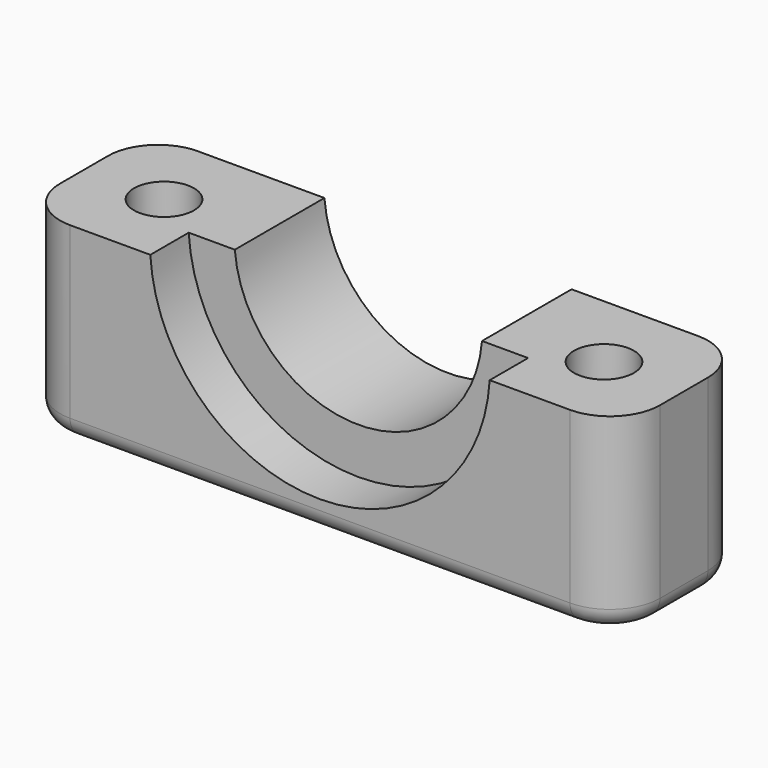
from build123d import *

# Parameters (mm, degrees)
F0_W         = 30
F0_H         = 8
F0_R         = 1.5
F1_DEPTH     = 10
F2_R         = 3.25
F2_R_2       = 1.5
F3_DEPTH     = 4
F5_DEPTH     = 8.001
F7_DEPTH     = 2.4
F8_R         = 2.5
F9_T1_DEPTH  = 3
F9_T3_DEPTH  = 25
F9_T6_ANGLE  = 90
F9_T8_ANGLE  = 90
F9_T10_ANGLE = 90
F9_T12_ANGLE = 90
F10_W        = 35.437501967
F10_H        = 11.6335232742
F10_R        = 1.5
F11_DEPTH    = 0.5


# Not quite as in the source:
# - a fillet or chamfer that OpenCascade refuses, or shapes differently, is made with other operations: its cross-section is extruded or revolved along the edge and cut away or added


with BuildPart() as f1:
    # F0 (on Top) → F1 (new body)
    with BuildSketch(Plane.XY):
        Rectangle(F0_W, F0_H)
        with Locations((-11, 0)):
            Circle(F0_R, mode=Mode.SUBTRACT)
        with Locations((11, 0)):
            Circle(F0_R, mode=Mode.SUBTRACT)
    extrude(amount=F1_DEPTH)

    # F2 (on face) → F3 (cut)
    with BuildSketch(Plane(origin=(0, 0, 0), x_dir=(1, 0, 0), z_dir=(0, 0, -1))):
        with Locations((11, 0)):
            Circle(F2_R)
        with Locations((11, 0)):
            Circle(F2_R_2, mode=Mode.SUBTRACT)
        with Locations((-11, 0)):
            Circle(F2_R)
        with Locations((-11, 0)):
            Circle(F2_R_2, mode=Mode.SUBTRACT)
    extrude(amount=-F3_DEPTH, mode=Mode.SUBTRACT)

    # F4 (on face) → F5 (cut, through all)
    with BuildSketch(Plane(origin=(0, 4, 0), x_dir=(-1, 0, 0), z_dir=(0, 1, 0))):
        with BuildLine():
            ThreePointArc((-6.2, 10), (0, 3.8), (6.2, 10))
            Line((6.2, 10), (-6.2, 10))
        make_face()
    extrude(amount=-F5_DEPTH, mode=Mode.SUBTRACT)

    # F6 (on face) → F7 (cut)
    with BuildSketch(Plane.XZ.offset(4)):
        with BuildLine():
            ThreePointArc((-8.5, 10), (0, 1.5), (8.5, 10))
            Line((8.5, 10), (6.2, 10))
            ThreePointArc((6.2, 10), (0, 3.8), (-6.2, 10))
            Line((-6.2, 10), (-8.5, 10))
        make_face()
    extrude(amount=-F7_DEPTH, mode=Mode.SUBTRACT)

    # F8
    f8_edges = [f1.edges().sort_by_distance(p)[0] for p in [
        (15, 4, 5),
        (15, -4, 5),
        (-15, 4, 5),
        (-15, -4, 5),
    ]]
    fillet(f8_edges, radius=F8_R)

    # F9: fillet of radius 1 on 8 edges, made by hand

    # F9_s2 → F9_t1 (cut)
    with BuildSketch(Plane.XZ.offset(-1.5)):
        with BuildLine():
            ThreePointArc((14, 0), (14.7071067812, 0.2928932188), (15, 1))
            Line((15, 1), (15, 0))
            Line((15, 0), (14, 0))
        make_face()
        with BuildLine():
            ThreePointArc((-14, 0), (-14.7071067812, 0.2928932188), (-15, 1))
            Line((-15, 1), (-15, 0))
            Line((-15, 0), (-14, 0))
        make_face()
    extrude(amount=F9_T1_DEPTH, mode=Mode.SUBTRACT)

    # F9_s4 → F9_t3 (cut)
    with BuildSketch(Plane.YZ.offset(-12.5)):
        with BuildLine():
            ThreePointArc((4, 1), (3.7071067812, 0.2928932188), (3, 0))
            Line((3, 0), (4, 0))
            Line((4, 0), (4, 1))
        make_face()
        with BuildLine():
            ThreePointArc((-3, 0), (-3.7071067812, 0.2928932188), (-4, 1))
            Line((-4, 1), (-4, 0))
            Line((-4, 0), (-3, 0))
        make_face()
    extrude(amount=F9_T3_DEPTH, mode=Mode.SUBTRACT)

    # F9_s5 → F9_t6 (revolve, cut)
    with BuildSketch(Plane.YZ.offset(12.5)):
        with BuildLine():
            ThreePointArc((3, 0), (3.7071067812, 0.2928932188), (4, 1))
            Line((4, 1), (4, 0))
            Line((4, 0), (3, 0))
        make_face()
    revolve(axis=Axis((12.5, 1.5, 0), (0, 0, -1)), revolution_arc=F9_T6_ANGLE, mode=Mode.SUBTRACT)

    # F9_s7 → F9_t8 (revolve, cut)
    with BuildSketch(Plane.YZ.offset(-12.5)):
        with BuildLine():
            ThreePointArc((3, 0), (3.7071067812, 0.2928932188), (4, 1))
            Line((4, 1), (4, 0))
            Line((4, 0), (3, 0))
        make_face()
    revolve(axis=Axis((-12.5, 1.5, 0), (0, 0, 1)), revolution_arc=F9_T8_ANGLE, mode=Mode.SUBTRACT)

    # F9_s9 → F9_t10 (revolve, cut)
    with BuildSketch(Plane.XZ.offset(1.5)):
        with BuildLine():
            ThreePointArc((14, 0), (14.7071067812, 0.2928932188), (15, 1))
            Line((15, 1), (15, 0))
            Line((15, 0), (14, 0))
        make_face()
    revolve(axis=Axis((12.5, -1.5, 0), (0, 0, -1)), revolution_arc=F9_T10_ANGLE, mode=Mode.SUBTRACT)

    # F9_s11 → F9_t12 (revolve, cut)
    with BuildSketch(Plane.XZ.offset(1.5)):
        with BuildLine():
            ThreePointArc((-14, 0), (-14.7071067812, 0.2928932188), (-15, 1))
            Line((-15, 1), (-15, 0))
            Line((-15, 0), (-14, 0))
        make_face()
    revolve(axis=Axis((-12.5, -1.5, 0), (0, 0, 1)), revolution_arc=F9_T12_ANGLE, mode=Mode.SUBTRACT)

    # F10 (on face) → F11 (cut)
    with BuildSketch(Plane.XY.offset(10)):
        with Locations((0.726422295, -0.4176155198)):
            Rectangle(F10_W, F10_H)
        with BuildLine():
            Line((12.5, -4), (8.5, -4))
            Line((8.5, -4), (8.5, -1.6))
            Line((8.5, -1.6), (6.2, -1.6))
            Line((6.2, -1.6), (6.2, 4))
            Line((6.2, 4), (12.5, 4))
            ThreePointArc((12.5, 4), (14.267766953, 3.267766953), (15, 1.5))
            Line((15, 1.5), (15, -1.5))
            ThreePointArc((15, -1.5), (14.267766953, -3.267766953), (12.5, -4))
        make_face(mode=Mode.SUBTRACT)
        with BuildLine():
            Line((8.5, -1.6), (8.5, -4))
            Line((8.5, -4), (12.5, -4))
            ThreePointArc((12.5, -4), (14.267766953, -3.267766953), (15, -1.5))
            Line((15, -1.5), (15, 1.5))
            ThreePointArc((15, 1.5), (14.267766953, 3.267766953), (12.5, 4))
            Line((12.5, 4), (6.2, 4))
            Line((6.2, 4), (6.2, -1.6))
            Line((6.2, -1.6), (8.5, -1.6))
        make_face()
        with Locations((11, 0)):
            Circle(F10_R, mode=Mode.SUBTRACT)
    extrude(amount=-F11_DEPTH, mode=Mode.SUBTRACT)


solid = f1.part
